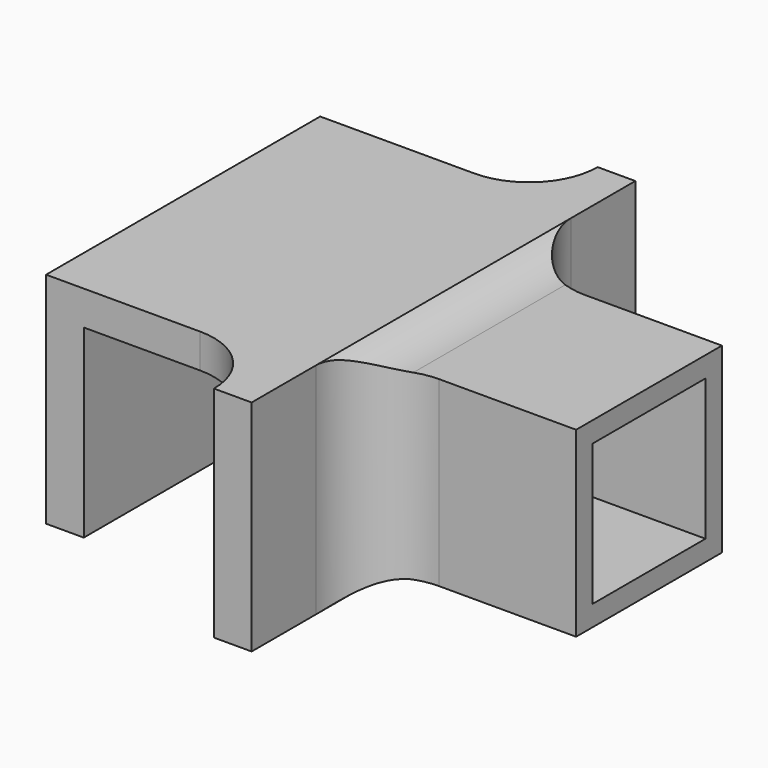
from build123d import *

# Parameters (mm, degrees)
F0_W         = 19
F0_H         = 25
F1_DEPTH     = 16
F2_W         = 13.5
F2_H         = 13.5011018194
F3_DEPTH     = 50
F4_W         = 5.15
F4_H         = 10.3
F5_DEPTH     = 2.75
F6_DEPTH     = 15
F7_T1_DEPTH  = 2.4988981806
F7_T3_DEPTH  = 13.2999992773
F7_T5_DEPTH  = 13.2999992773
F7_T11_DEPTH = 21.6634917276
F7_T15_DEPTH = 25.7999992773
F7_T23_DEPTH = 21.6634917276
F7_T27_DEPTH = 25.7999992773
F7_T35_DEPTH = 22.0158699277
F7_T39_DEPTH = 25.7999992773
F7_T47_DEPTH = 25.7999992773
F7_T52_DEPTH = 22.0158699277


# Not quite as in the source:
# - a fillet or chamfer that OpenCascade refuses, or shapes differently, is made with other operations: its cross-section is extruded or revolved along the edge and cut away or added
# - a feature names something its author has since deleted; it is built from what else it names


with BuildPart() as f1:
    # F0 (on Top) → F1 (new body)
    with BuildSketch(Plane.XY):
        Rectangle(F0_W, F0_H)
    extrude(amount=F1_DEPTH)

    # F2 (on face) → F3 (cut)
    with BuildSketch(Plane.XZ.offset(12.5)):
        with Locations((0, 6.7505509097)):
            Rectangle(F2_W, F2_H)
    extrude(amount=-F3_DEPTH, mode=Mode.SUBTRACT)

    # F4 (on face) → F5 (join)
    with BuildSketch(Plane.YZ.offset(9.5)):
        Polygon((0, 16), (-17.5, 16), (-17.5, 0), (0, 0), (0, 1.4159553841), (-6.6499996386, 1.4159553841), (-6.6499996386, 14.7159546614), (0, 14.7159546614), align=None)
        Polygon((17.5, 16), (0, 16), (0, 14.7159546614), (6.6499996386, 14.7159546614), (6.6499996386, 1.4159553841), (0, 1.4159553841), (0, 0), (17.5, 0), align=None)
        with Locations((-2.575, 8.0659550227)):
            Rectangle(F4_W, F4_H)
        with Locations((2.575, 8.0659550227)):
            Rectangle(F4_W, F4_H)
        Polygon((0, 13.2159550227), (0, 14.7159546614), (-6.6499996386, 14.7159546614), (-6.6499996386, 1.4159553841), (0, 1.4159553841), (0, 2.9159550227), (-5.15, 2.9159550227), (-5.15, 13.2159550227), align=None)
        Polygon((6.6499996386, 14.7159546614), (0, 14.7159546614), (0, 13.2159550227), (5.15, 13.2159550227), (5.15, 2.9159550227), (0, 2.9159550227), (0, 1.4159553841), (6.6499996386, 1.4159553841), align=None)
    extrude(amount=-F5_DEPTH)

    # F4 (on face) → F6 (join)
    with BuildSketch(Plane.YZ.offset(9.5)):
        Polygon((0, 13.2159550227), (0, 14.7159546614), (-6.6499996386, 14.7159546614), (-6.6499996386, 1.4159553841), (0, 1.4159553841), (0, 2.9159550227), (-5.15, 2.9159550227), (-5.15, 13.2159550227), align=None)
        Polygon((6.6499996386, 14.7159546614), (0, 14.7159546614), (0, 13.2159550227), (5.15, 13.2159550227), (5.15, 2.9159550227), (0, 2.9159550227), (0, 1.4159553841), (6.6499996386, 1.4159553841), align=None)
    extrude(amount=F6_DEPTH)

    # F7: fillet of radius 5 on 6 edges, made by hand

    # F7_s2 → F7_t1 (join)
    with BuildSketch(Plane.XY.offset(13.5011018194)):
        with BuildLine():
            ThreePointArc((6.75, 17.5), (5.2855339059, 13.9644660941), (1.75, 12.5))
            Line((1.75, 12.5), (6.75, 12.5))
            Line((6.75, 12.5), (6.75, 17.5))
        make_face()
        with BuildLine():
            ThreePointArc((6.75, -17.5), (5.2855339059, -13.9644660941), (1.75, -12.5))
            Line((1.75, -12.5), (6.75, -12.5))
            Line((6.75, -12.5), (6.75, -17.5))
        make_face()
    extrude(amount=F7_T1_DEPTH)

    # F7_s4 → F7_t3 (join)
    with BuildSketch(Plane.XZ.offset(-6.6499996386)):
        with BuildLine():
            ThreePointArc((9.5, 16), (11.0537180617, 15.0479907955), (12.8453969801, 14.7159546614))
            Line((12.8453969801, 14.7159546614), (9.5, 14.7159546614))
            Line((9.5, 14.7159546614), (9.5, 16))
        make_face()
        with BuildLine():
            ThreePointArc((9.5, 0), (11.1048891295, 1.0484613517), (12.9863482602, 1.4159553841))
            Line((12.9863482602, 1.4159553841), (9.5, 1.4159553841))
            Line((9.5, 1.4159553841), (9.5, 0))
        make_face()
    extrude(amount=F7_T3_DEPTH)

    # F7_s6 → F7_t5 (join)
    with BuildSketch(Plane.XY.offset(1.4159553841)):
        with BuildLine():
            ThreePointArc((9.5, -11.6499996386), (10.9644660941, -8.1144657327), (14.5, -6.6499996386))
            Line((14.5, -6.6499996386), (9.5, -6.6499996386))
            Line((9.5, -6.6499996386), (9.5, -11.6499996386))
        make_face()
        with BuildLine():
            ThreePointArc((9.5, 11.6499996386), (10.9644660941, 8.1144657327), (14.5, 6.6499996386))
            Line((14.5, 6.6499996386), (9.5, 6.6499996386))
            Line((9.5, 6.6499996386), (9.5, 11.6499996386))
        make_face()
    extrude(amount=F7_T5_DEPTH)


with BuildPart() as f7_tool9:
    # F7_s10 → F7_t11 (new body)
    with BuildSketch(Plane.XZ.offset(-15.013492089)):
        with BuildLine():
            ThreePointArc((9.5, 16), (11.0537180617, 15.0479907955), (12.8453969801, 14.7159546614))
            Line((12.8453969801, 14.7159546614), (9.5, 14.7159546614))
            Line((9.5, 14.7159546614), (9.5, 16))
        make_face()
    extrude(amount=F7_T11_DEPTH)

    split(bisect_by=Plane.XZ.offset(-6.6499996386), keep=Keep.BOTTOM)


with BuildPart() as f7_tool13:
    # F7_s14 → F7_t15 (new body)
    with BuildSketch(Plane.XY.offset(1.4159553841)):
        with BuildLine():
            ThreePointArc((9.5, 11.6499996386), (10.9644660941, 8.1144657327), (14.5, 6.6499996386))
            Line((14.5, 6.6499996386), (9.5, 6.6499996386))
            Line((9.5, 6.6499996386), (9.5, 11.6499996386))
        make_face()
    extrude(amount=F7_T15_DEPTH)

    split(bisect_by=Plane.XY.offset(16), keep=Keep.BOTTOM)

    split(bisect_by=Plane.XY.offset(14.7159546614), keep=Keep.TOP)


with BuildPart() as f7_tool9_1:
    add(f7_tool9.part)

    # F7_t18: intersect F7_tool13
    add(f7_tool13.part, mode=Mode.INTERSECT)


with BuildPart() as f1_1:
    add(f1.part)

    # F7_t7: union F7_tool9
    add(f7_tool9_1.part)


with BuildPart() as f7_tool21:
    # F7_s22 → F7_t23 (new body)
    with BuildSketch(Plane.XZ.offset(-6.6499996386)):
        with BuildLine():
            ThreePointArc((9.5, 16), (11.0537180617, 15.0479907955), (12.8453969801, 14.7159546614))
            Line((12.8453969801, 14.7159546614), (9.5, 14.7159546614))
            Line((9.5, 14.7159546614), (9.5, 16))
        make_face()
    extrude(amount=F7_T23_DEPTH)

    split(bisect_by=Plane.XZ.offset(6.6499996386), keep=Keep.TOP)


with BuildPart() as f7_tool25:
    # F7_s26 → F7_t27 (new body)
    with BuildSketch(Plane.XY.offset(27.2159546614)):
        with BuildLine():
            ThreePointArc((9.5, -11.6499996386), (10.9644660941, -8.1144657327), (14.5, -6.6499996386))
            Line((14.5, -6.6499996386), (9.5, -6.6499996386))
            Line((9.5, -6.6499996386), (9.5, -11.6499996386))
        make_face()
    extrude(amount=-F7_T27_DEPTH)

    split(bisect_by=Plane.XY.offset(16), keep=Keep.BOTTOM)

    split(bisect_by=Plane.XY.offset(14.7159546614), keep=Keep.TOP)


with BuildPart() as f7_tool21_1:
    add(f7_tool21.part)

    # F7_t30: intersect F7_tool25
    add(f7_tool25.part, mode=Mode.INTERSECT)


with BuildPart() as f1_2:
    add(f1_1.part)

    # F7_t19: union F7_tool21
    add(f7_tool21_1.part)


with BuildPart() as f7_tool33:
    # F7_s34 → F7_t35 (new body)
    with BuildSketch(Plane.XZ.offset(15.365870289)):
        with BuildLine():
            ThreePointArc((9.5, 0), (11.1048891295, 1.0484613517), (12.9863482602, 1.4159553841))
            Line((12.9863482602, 1.4159553841), (9.5, 1.4159553841))
            Line((9.5, 1.4159553841), (9.5, 0))
        make_face()
    extrude(amount=-F7_T35_DEPTH)

    split(bisect_by=Plane.XZ.offset(6.6499996386), keep=Keep.TOP)


with BuildPart() as f7_tool37:
    # F7_s38 → F7_t39 (new body)
    with BuildSketch(Plane.XY.offset(14.7159546614)):
        with BuildLine():
            ThreePointArc((9.5, -11.6499996386), (10.9644660941, -8.1144657327), (14.5, -6.6499996386))
            Line((14.5, -6.6499996386), (9.5, -6.6499996386))
            Line((9.5, -6.6499996386), (9.5, -11.6499996386))
        make_face()
    extrude(amount=-F7_T39_DEPTH)

    split(bisect_by=Plane.XY, keep=Keep.TOP)

    split(bisect_by=Plane.XY.offset(1.4159553841), keep=Keep.BOTTOM)


with BuildPart() as f7_tool33_1:
    add(f7_tool33.part)

    # F7_t42: intersect F7_tool37
    add(f7_tool37.part, mode=Mode.INTERSECT)


with BuildPart() as f1_3:
    add(f1_2.part)

    # F7_t31: union F7_tool33
    add(f7_tool33_1.part)


with BuildPart() as f7_tool45:
    # F7_s46 → F7_t47 (new body)
    with BuildSketch(Plane.XY.offset(-11.0840446159)):
        with BuildLine():
            ThreePointArc((9.5, 11.6499996386), (10.9644660941, 8.1144657327), (14.5, 6.6499996386))
            Line((14.5, 6.6499996386), (9.5, 6.6499996386))
            Line((9.5, 6.6499996386), (9.5, 11.6499996386))
        make_face()
    extrude(amount=F7_T47_DEPTH)

    split(bisect_by=Plane.XY, keep=Keep.TOP)

    split(bisect_by=Plane.XY.offset(1.4159553841), keep=Keep.BOTTOM)


with BuildPart() as f7_tool50:
    # F7_s51 → F7_t52 (new body)
    with BuildSketch(Plane.XZ.offset(6.6499996386)):
        with BuildLine():
            ThreePointArc((9.5, 0), (11.1048891295, 1.0484613517), (12.9863482602, 1.4159553841))
            Line((12.9863482602, 1.4159553841), (9.5, 1.4159553841))
            Line((9.5, 1.4159553841), (9.5, 0))
        make_face()
    extrude(amount=-F7_T52_DEPTH)

    split(bisect_by=Plane.XZ.offset(-6.6499996386), keep=Keep.BOTTOM)


with BuildPart() as f7_tool45_1:
    add(f7_tool45.part)

    # F7_t54: intersect F7_tool50
    add(f7_tool50.part, mode=Mode.INTERSECT)


with BuildPart() as f1_4:
    add(f1_3.part)

    # F7_t43: union F7_tool45
    add(f7_tool45_1.part)


solid = f1_4.part
